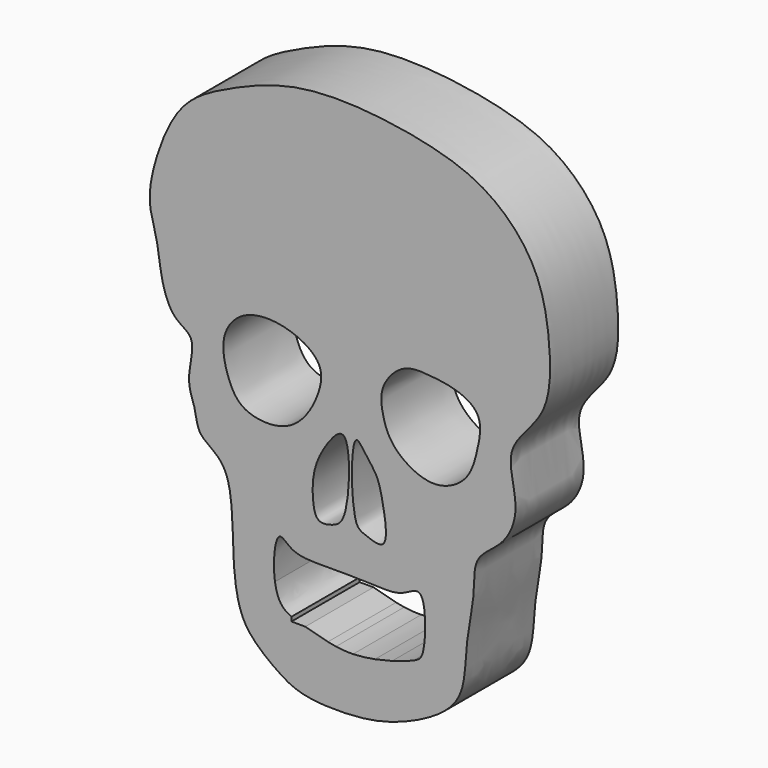
from build123d import *

# Parameters (mm, degrees)
F1_DEPTH = 17.78


# Not quite as in the source:
# - the program builds the solid bodies; features that only make, move or delete a surface that nothing else refers to are left out


with BuildPart() as f1:
    # F0 (on Front) → F1 (new body)
    with BuildSketch(Plane.XZ):
        with BuildLine():
            add(Edge.make_bspline(
                [(-20.9226347506, -71.2602362037), (-22.9886342213, -70.7506123091), (-26.0301044902, -69.0380612745), (-31.1666456634, -65.0505667557), (-34.2689378028, -60.6176976927), (-35.5822291113, -52.2647973285), (-35.4627694042, -42.6269395546), (-36.8498794394, -33.613895217), (-43.0496971354, -30.9908814125), (-43.1466641232, -26.0636418667), (-45.6318612712, -21.4562205965), (-42.723481771, -13.0323540897), (-48.1701631476, -11.4026865835), (-50.6596581538, -4.5826420913), (-51.1570706347, 2.5334279955), (-53.6932475631, 8.8560882656), (-51.2546569538, 19.164436079), (-46.4065160275, 29.6700504939), (-36.5811839124, 35.0025530943), (-23.1580005213, 40.489791694), (-7.7072946703, 40.4727885367), (6.4712539836, 38.1512957348), (18.1604650619, 34.1017346949), (28.4147710656, 23.6174553255), (30.911400155, 9.4088083889), (30.6728119611, -4.1893708351), (20.2242742309, -11.8090645901), (24.8010252062, -22.4800291026), (21.1053201708, -30.6111839492), (14.4097792293, -34.0465505235), (15.0828088795, -41.7123951546), (12.8857178127, -50.3397512226), (13.0649687999, -60.6633470175), (7.2854967108, -66.4298943527), (-2.3574186317, -70.8167790943), (-10.982688846, -72.1394021849), (-18.2300625399, -71.92441795), (-20.9226347506, -71.2602362037)],
                knots=[0, 0, 0, 0, 0.0228917331, 0.0468708008, 0.0688593266, 0.0962849122, 0.1268675457, 0.1548243145, 0.1777038778, 0.1975208964, 0.2195912859, 0.2457564995, 0.2656295096, 0.290732991, 0.3165181546, 0.3409929532, 0.3717694787, 0.403982822, 0.4354354186, 0.4718026973, 0.5095410579, 0.5458342986, 0.5792879041, 0.614900291, 0.6512466949, 0.685711094, 0.7173188118, 0.7475903097, 0.7751031966, 0.7997793498, 0.8247034334, 0.8538976743, 0.883972496, 0.9103832483, 0.9412228343, 0.9701657017, 1, 1, 1, 1], degree=3))
        make_face()
        with BuildLine():
            add(Edge.make_bspline(
                [(-12.4493716285, -21.0603736341), (-10.829230374, -22.3302554562), (-11.1915395304, -36.4652533596), (-14.4835500635, -38.2509141163), (-18.1705359121, -39.0157648002), (-19.0142803498, -34.7090389314), (-18.8817734758, -29.3196721187), (-16.5854441236, -24.2821601952), (-13.3519027008, -20.3529613641), (-12.4493716285, -21.0603736341)],
                knots=[0, 0, 0, 0, 0.2336678543, 0.3535085639, 0.4560029301, 0.5717415004, 0.7155303715, 0.869830795, 1, 1, 1, 1], degree=3))
        make_face(mode=Mode.SUBTRACT)
        with BuildLine():
            add(Edge.make_bspline(
                [(-25.876455009, -43.9899750054), (-26.8082138316, -44.681997323), (-27.2755063744, -49.0720417723), (-26.7589227771, -52.5409724782)],
                knots=[0, 0, 0, 0, 0.0880237985, 0.0880237985, 0.0880237985, 0.0880237985], degree=3))
            add(Edge.make_bspline(
                [(-23.3194921166, -45.3258417547), (-24.4662885556, -44.6564309517), (-25.2698138816, -43.5394193587), (-25.876455009, -43.9899750054)],
                knots=[0.9426902595, 0.9426902595, 0.9426902595, 0.9426902595, 1, 1, 1, 1], degree=3))
            add(Edge.make_bspline(
                [(-20.4180553555, -46.1791414835), (-21.5174121124, -46.0509177156), (-22.5050249683, -45.8012644968), (-23.3194921166, -45.3258417547)],
                knots=[0.9019882662, 0.9019882662, 0.9019882662, 0.9019882662, 0.9426902595, 0.9426902595, 0.9426902595, 0.9426902595], degree=3))
            add(Edge.make_bspline(
                [(-15.7204885036, -46.2929904461), (-17.3847926735, -46.3076350432), (-18.9950372744, -46.345115576), (-20.4180553555, -46.1791414835)],
                knots=[0.8493032102, 0.8493032102, 0.8493032102, 0.8493032102, 0.9019882662, 0.9019882662, 0.9019882662, 0.9019882662], degree=3))
            add(Edge.make_bspline(
                [(-10.7723470241, -46.309964849), (-12.4069148876, -46.286216951), (-14.0896552183, -46.278640367), (-15.7204885036, -46.2929904461)],
                knots=[0.7976777053, 0.7976777053, 0.7976777053, 0.7976777053, 0.8493032102, 0.8493032102, 0.8493032102, 0.8493032102], degree=3))
            add(Edge.make_bspline(
                [(-5.9108668938, -46.4311540127), (-7.4019328535, -46.3774312878), (-9.060729449, -46.3348321674), (-10.7723470241, -46.309964849)],
                knots=[0.7436186947, 0.7436186947, 0.7436186947, 0.7436186947, 0.7976777053, 0.7976777053, 0.7976777053, 0.7976777053], degree=3))
            add(Edge.make_bspline(
                [(-2.3311186086, -46.4311540127), (-3.4305119234, -46.5336573619), (-4.6065123191, -46.4781495742), (-5.9108668938, -46.4311540127)],
                knots=[0.6963289573, 0.6963289573, 0.6963289573, 0.6963289573, 0.7436186947, 0.7436186947, 0.7436186947, 0.7436186947], degree=3))
            add(Edge.make_bspline(
                [(4.5037194588, -52.5409724782), (4.7062271291, -49.5633453673), (4.3281969185, -42.8215296425), (0.6657290389, -45.8961991189), (-1.5192487102, -46.3554582788), (-2.3311186086, -46.4311540127)],
                knots=[0.5163609284, 0.5163609284, 0.5163609284, 0.5163609284, 0.5972448361, 0.6614068654, 0.6963289573, 0.6963289573, 0.6963289573, 0.6963289573], degree=3))
            add(Edge.make_bspline(
                [(2.1026290487, -57.6224140823), (3.3605482708, -57.0718606927), (4.0653451976, -56.4884533312), (4.4357999194, -53.5396460666), (4.5037194588, -52.5409724782)],
                knots=[0.4285239488, 0.4285239488, 0.4285239488, 0.4285239488, 0.4892330782, 0.5163609284, 0.5163609284, 0.5163609284, 0.5163609284], degree=3))
            add(Edge.make_bspline(
                [(-2.3311186086, -59.1451756831), (-0.5215999354, -58.639628573), (1.0568718328, -58.0801105463), (2.1026290487, -57.6224140823)],
                knots=[0.3780540863, 0.3780540863, 0.3780540863, 0.3780540863, 0.4285239488, 0.4285239488, 0.4285239488, 0.4285239488], degree=3))
            add(Edge.make_bspline(
                [(-5.9108668938, -59.9898483283), (-4.6765560372, -59.7544057168), (-3.4589587425, -59.4602740177), (-2.3311186086, -59.1451756831)],
                knots=[0.3465971374, 0.3465971374, 0.3465971374, 0.3465971374, 0.3780540863, 0.3780540863, 0.3780540863, 0.3780540863], degree=3))
            add(Edge.make_bspline(
                [(-10.4702683166, -60.5238489807), (-9.0191975358, -60.4862931551), (-7.4520043668, -60.2838175739), (-5.9108668938, -59.9898483283)],
                knots=[0.3073205788, 0.3073205788, 0.3073205788, 0.3073205788, 0.3465971374, 0.3465971374, 0.3465971374, 0.3465971374], degree=3))
            add(Edge.make_bspline(
                [(-14.0320396464, -60.2961386998), (-12.9192111237, -60.4634255551), (-11.7391354352, -60.55668911), (-10.4702683166, -60.5238489807)],
                knots=[0.2729757802, 0.2729757802, 0.2729757802, 0.2729757802, 0.3073205788, 0.3073205788, 0.3073205788, 0.3073205788], degree=3))
            add(Edge.make_bspline(
                [(-15.7204885036, -59.9815773863), (-15.1739097224, -60.1016265638), (-14.612110549, -60.2089390683), (-14.0320396464, -60.2961386998)],
                knots=[0.255073275, 0.255073275, 0.255073275, 0.255073275, 0.2729757802, 0.2729757802, 0.2729757802, 0.2729757802], degree=3))
            add(Edge.make_bspline(
                [(-20.4180553555, -58.7277188897), (-18.9369313978, -59.1231916021), (-17.4006176954, -59.6125580708), (-15.7204885036, -59.9815773863)],
                knots=[0.2000427423, 0.2000427423, 0.2000427423, 0.2000427423, 0.255073275, 0.255073275, 0.255073275, 0.255073275], degree=3))
            Line((-20.4180553555, -58.7277188897), (-23.3194921166, -58.7277188897))
            Line((-23.3194921166, -58.7277188897), (-23.3194921166, -57.8472660991))
            add(Edge.make_bspline(
                [(-26.7589227771, -52.5409724782), (-26.6143701808, -53.5116632674), (-25.9474677782, -56.2159884416), (-24.4796867279, -57.3503153053), (-23.3194921166, -57.8472660991)],
                knots=[0.0880237985, 0.0880237985, 0.0880237985, 0.0880237985, 0.1126549882, 0.162153843, 0.162153843, 0.162153843, 0.162153843], degree=3))
        make_face(mode=Mode.SUBTRACT)
        with BuildLine():
            add(Edge.make_bspline(
                [(-9.8674017936, -21.0603736341), (-11.0128428563, -22.0880001403), (-10.8790656481, -36.7722003639), (-8.2158939088, -37.6567846761), (-2.6795293613, -39.9587056149), (-4.2808324195, -30.5470254811), (-5.2369907779, -26.0992788001), (-7.8254242786, -23.1973871392), (-9.3947137725, -20.6363040286), (-9.8674017936, -21.0603736341)],
                knots=[0, 0, 0, 0, 0.2379415243, 0.3470800591, 0.465777058, 0.6340254385, 0.7745140926, 0.9018089085, 1, 1, 1, 1], degree=3))
        make_face(mode=Mode.SUBTRACT)
        with BuildLine():
            add(Edge.make_bspline(
                [(-17.6133103669, -9.6259368584), (-16.7915361215, -11.2202701541), (-17.4272897806, -15.0859816115), (-20.4199107518, -20.7332219768), (-25.3764034964, -24.4421930464), (-33.8271124958, -23.752448571), (-36.8038646033, -18.1105419651), (-38.3787688337, -10.9229876004), (-33.630003342, -4.526506425), (-24.2048522234, -4.4067552806), (-18.6225326828, -7.6679334892), (-17.6133103669, -9.6259368584)],
                knots=[0, 0, 0, 0, 0.0978086176, 0.2050040575, 0.3089201047, 0.4251497023, 0.5286364792, 0.641223732, 0.7522135924, 0.8798810743, 1, 1, 1, 1], degree=3))
        make_face(mode=Mode.SUBTRACT)
        with BuildLine():
            add(Edge.make_bspline(
                [(-4.2423959821, -9.6259368584), (-4.7997731181, -11.2996363883), (-4.3623758823, -14.4298950921), (-3.0777807037, -18.6166996651), (0.7398538249, -22.3572914891), (7.0327110981, -24.7413735393), (13.7104948343, -21.1560833864), (15.4505862881, -14.9820605467), (16.7838233922, -8.1076566408), (11.790477128, -4.9266573903), (5.750541843, -4.1132888004), (-0.2852097044, -3.7491609516), (-3.5948628732, -7.681515765), (-4.2423959821, -9.6259368584)],
                knots=[0, 0, 0, 0, 0.0832317834, 0.1614126581, 0.2476828932, 0.3433370881, 0.4412803885, 0.5374774647, 0.6327029315, 0.717549293, 0.8122148935, 0.9033054426, 1, 1, 1, 1], degree=3))
        make_face(mode=Mode.SUBTRACT)
    extrude(amount=F1_DEPTH)


solid = f1.part
